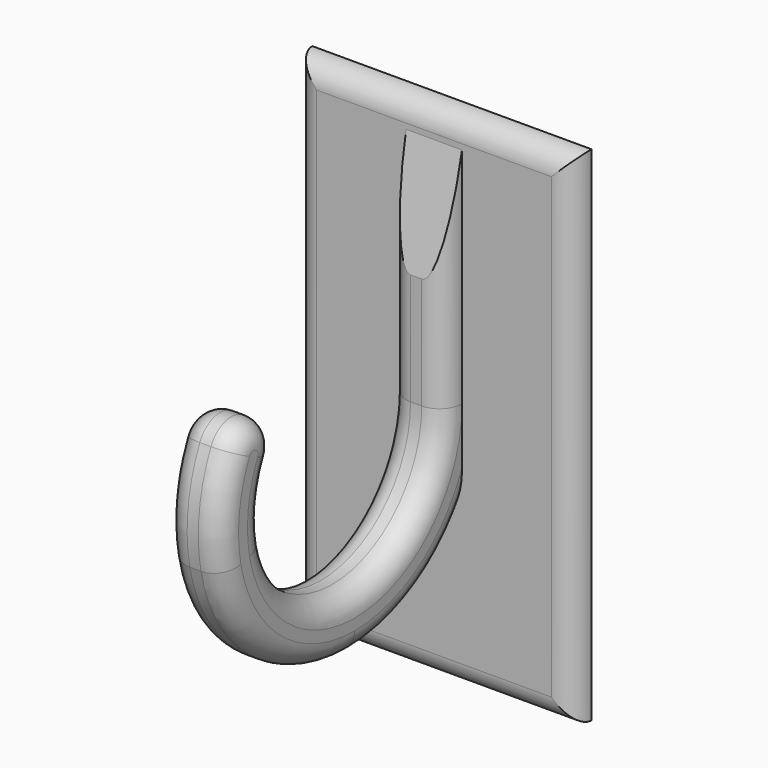
from build123d import *

# Parameters (mm, degrees)
F0_W     = 25
F0_H     = 45
F1_DEPTH = 2
F2_W     = 5
F2_H     = 35
F3_DEPTH = 50
F5_DEPTH = 5
F6_R     = 1.99999


# Not quite as in the source:
# - a fillet or chamfer is up to 0.001 mm smaller than in the source, because OpenCascade refuses the exact size


with BuildPart() as f1:
    # F0 (on Front) → F1 (new body)
    with BuildSketch(Plane.XZ):
        Rectangle(F0_W, F0_H)
    extrude(amount=F1_DEPTH)

    # F2 (on face) → F3 (join)
    with BuildSketch(Plane.XZ.offset(2)):
        with Locations((0, 2.5)):
            Rectangle(F2_W, F2_H)
    extrude(amount=F3_DEPTH)

    # F4 (on face) → F5 (cut, through all)
    with BuildSketch(Plane.YZ.offset(2.5)):
        with BuildLine():
            Line((-4, 10), (-2, 20))
            Line((-2, 20), (-52, 20))
            Line((-52, 20), (-52, -15))
            Line((-52, -15), (-14.0000000101, -15))
            ThreePointArc((-14.0000000101, -15), (-23.4927752917, -11.6140956282), (-28.7, -2.9849623113))
            ThreePointArc((-28.7, -2.9849623113), (-28.8931709496, 1.7870252), (-27.5765596133, 6.3778545818))
            ThreePointArc((-27.5765596133, 6.3778545818), (-24.2508239141, 7.5776387537), (-23.0510397422, 4.2519030545))
            ThreePointArc((-23.0510397422, 4.2519030545), (-23.9287806331, 1.1913501333), (-23.8, -1.9899748742))
            ThreePointArc((-23.8, -1.9899748742), (-13, -9.9498743711), (-4, 0))
            Line((-4, 0), (-4, 10))
        make_face()
        with BuildLine():
            Line((-2, -15), (-2, -9))
            ThreePointArc((-2, -9), (-7.291796072, -13.4164078673), (-14.0000000101, -15))
            Line((-14.0000000101, -15), (-2, -15))
        make_face()
    extrude(amount=-F5_DEPTH, mode=Mode.SUBTRACT)

    # F6 (radius 2 in the source; OpenCascade refuses exactly that, so slightly less here)
    f6_edges = [f1.edges().sort_by_distance(p)[0] for p in [
        (2.5, -24.250824, 7.577639),
        (-2.5, -24.250824, 7.577639),
        (0, -2, 22.5),
        (-12.5, -2, 0),
        (0, -2, -22.5),
        (12.5, -2, 0),
    ]]
    fillet(f6_edges, radius=F6_R)


solid = f1.part
